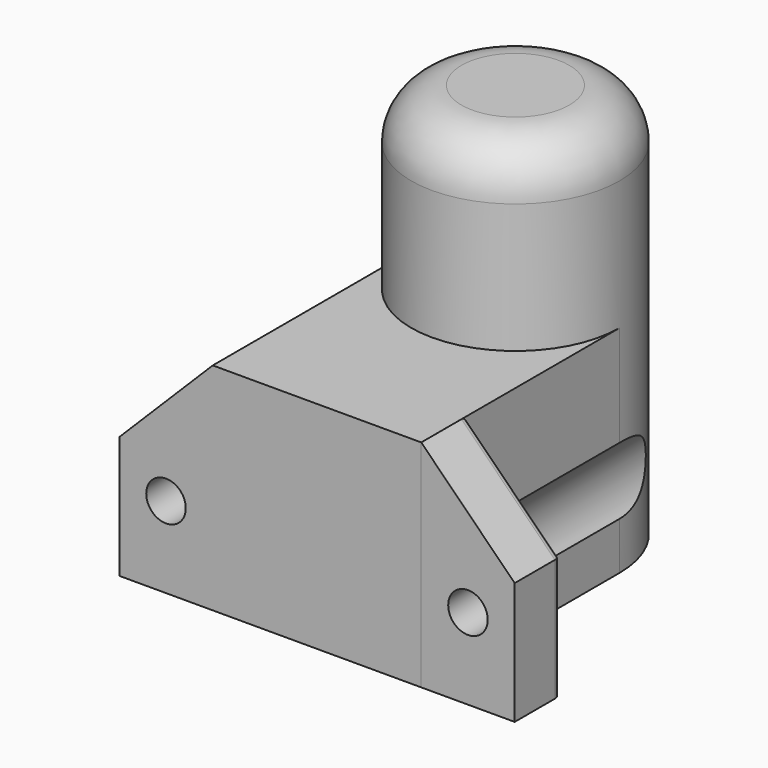
from build123d import *

# Parameters (mm, degrees)
F0_W      = 49
F0_H      = 30
F1_DEPTH  = 29
F3_DEPTH  = 8
F5_DEPTH  = 25
F6_DEPTH  = 30
F8_R      = 2.75
F9_DEPTH  = 25
F10_R     = 8
F11_DEPTH = 40
F12_R     = 1
F12_2_R   = 1


# Not quite as in the source:
# - a fillet or chamfer that OpenCascade refuses, or shapes differently, is made with other operations: its cross-section is extruded or revolved along the edge and cut away or added


with BuildPart() as f1:
    # F0 (on Right) → F1 (new body)
    with BuildSketch(Plane.YZ):
        with Locations((24.5, 15)):
            Rectangle(F0_W, F0_H)
    extrude(amount=F1_DEPTH)

    # F2 (on Front) → F3 (join)
    with BuildSketch(Plane.XZ):
        Polygon((-13, 0), (0, 0), (0, 30), (-13, 17), align=None)
    extrude(amount=-F3_DEPTH)

    # F4 (on face) → F5 (join)
    with BuildSketch(Plane.XY.offset(30)):
        with BuildLine():
            ThreePointArc((29, 34.5), (24.7530483272, 44.7530483272), (14.5, 49))
            Line((14.5, 49), (14.5, 20))
            ThreePointArc((14.5, 20), (24.7530483272, 24.2469516728), (29, 34.5))
        make_face()
        with BuildLine():
            Line((14.5, 20), (14.5, 49))
            ThreePointArc((14.5, 49), (0, 34.5), (14.5, 20))
        make_face()
    extrude(amount=F5_DEPTH)

    # F6 (cut): faces of the model
    f6_faces = [f1.faces().sort_by_distance(p)[0] for p in [
        (25.7611648853, 45.7611648853, 30),
        (3.2388351147, 45.7611648853, 30),
    ]]
    extrude(f6_faces, amount=-F6_DEPTH, mode=Mode.SUBTRACT)

    # F7: fillet of radius 7 on 1 edges, made by hand

    # F7_s1 → F7_t2 (revolve, cut)
    with BuildSketch(Plane.XZ.offset(-34.5)):
        with BuildLine():
            ThreePointArc((29, 48), (26.9497474683, 52.9497474683), (22, 55))
            Line((22, 55), (29, 55))
            Line((29, 55), (29, 48))
        make_face()
    revolve(axis=Axis((14.5, 34.5, 55), (0, 0, 1)), mode=Mode.SUBTRACT)


with BuildPart() as f3:
    # F2 (on Front) → F3, piece 2 (new body)
    with BuildSketch(Plane.XZ):
        Polygon((29.0028285235, 30), (29.0028285235, 0), (42.0028285235, 0), (42.0028285235, 17), align=None)
    extrude(amount=-F3_DEPTH)


with BuildPart() as f9_tool:
    # F8 (on face) → F9 (new body)
    with BuildSketch(Plane(origin=(0, 8, 0), x_dir=(-1, 0, 0), z_dir=(0, 1, 0))):
        with Locations((-35.5028285235, 11.2820267677)):
            Circle(F8_R)
        with Locations((6.5, 11.2820267677)):
            Circle(F8_R)
    extrude(amount=-F9_DEPTH)


with BuildPart() as f1_1:
    add(f1.part)

    # F9: cut by f9_tool
    add(f9_tool.part, mode=Mode.SUBTRACT)

    # F10 (on face) → F11 (cut)
    with BuildSketch(Plane(origin=(0, 8, 0), x_dir=(-1, 0, 0), z_dir=(0, 1, 0))):
        with Locations((-35.5028285235, 11.2820267677)):
            Circle(F10_R)
        with Locations((6.708932967, 11.5158854604)):
            Circle(F10_R)
    extrude(amount=F11_DEPTH, mode=Mode.SUBTRACT)

    # F12
    f12_edges = [f1_1.edges().sort_by_distance(p)[0] for p in [
        (-6.5, 8, 23.5),
        (-13, 8, 8.5),
    ]]
    fillet(f12_edges, radius=F12_R)


with BuildPart() as f3_1:
    add(f3.part)

    # F9: cut by f9_tool
    add(f9_tool.part, mode=Mode.SUBTRACT)

    # F12#2
    f12_2_edges = [f3_1.edges().sort_by_distance(p)[0] for p in [
        (35.502829, 8, 23.5),
        (42.002829, 8, 8.5),
    ]]
    fillet(f12_2_edges, radius=F12_2_R)


solid = Compound([f1_1.part, f3_1.part])
